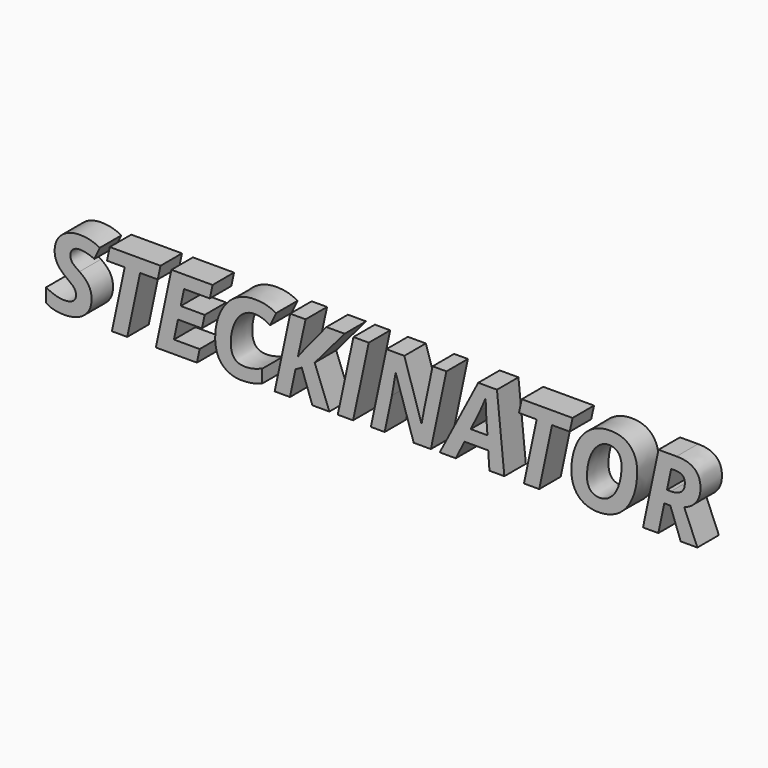
from build123d import *

# Parameters (mm, degrees)
F0_TEXT_SIZE = 11.5045491205
F1_DEPTH     = 3


# Not quite as in the source:
# - Text() gives the source's letters only with a copy of the font that has no kerning and outlines rounded to 1/6400 em; it was checked with that copy


with BuildPart() as f1:
    # F0 (on Front) → F1 (new body)
    with BuildSketch(Plane.XZ):
        with Locations((-74.1072721941, 0)):
            Text('STECKINATOR', F0_TEXT_SIZE, font='Open Sans', font_style=FontStyle.BOLDITALIC, text_align=(TextAlign.LEFT, TextAlign.BOTTOM))
    extrude(amount=F1_DEPTH)


solid = f1.part
